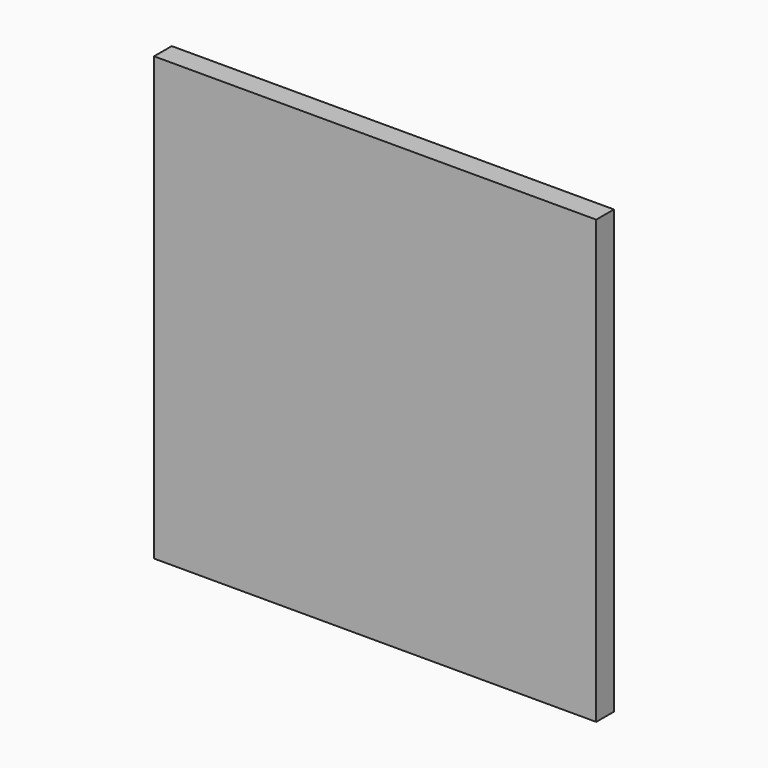
from build123d import *

# Parameters (mm, degrees)
F0_W     = 100
F0_H     = 100
F1_DEPTH = 5


with BuildPart() as f1:
    # F0 (on Front) → F1 (new body)
    with BuildSketch(Plane.XZ):
        with Locations((225, 50)):
            Rectangle(F0_W, F0_H)
    extrude(amount=F1_DEPTH)


solid = f1.part
